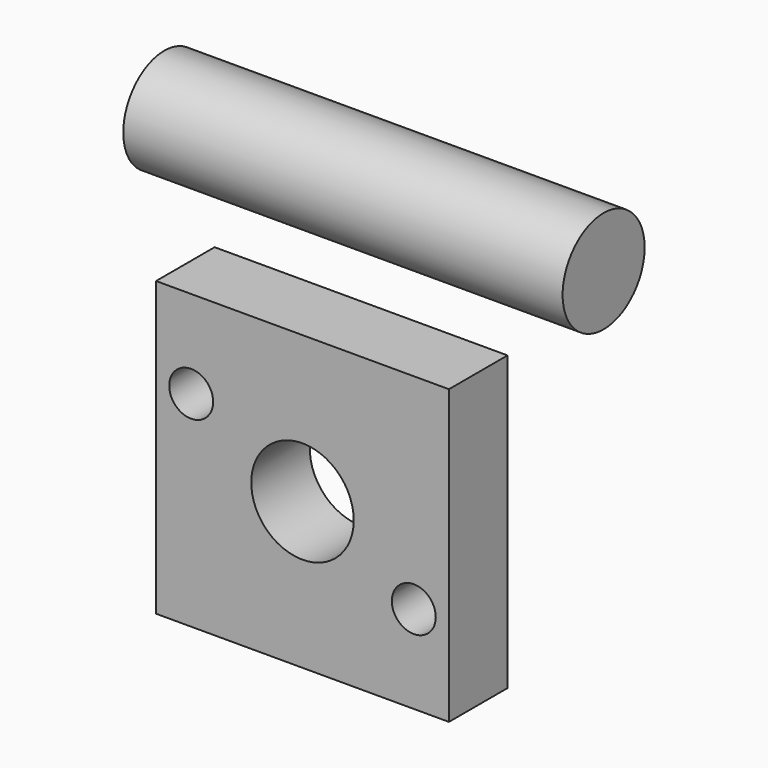
from build123d import *

# Parameters (mm, degrees)
F0_W     = 100
F0_H     = 100
F0_R     = 7.5
F0_R_2   = 17.5
F1_DEPTH = 25
F2_R     = 17.5
F3_DEPTH = 150
F4_R     = 7.5
F5_DEPTH = 5
F6_R     = 7.5
F7_DEPTH = 146.0218702087


with BuildPart() as f1:
    # F0 (on Front) → F1 (new body)
    with BuildSketch(Plane.XZ):
        Rectangle(F0_W, F0_H)
        with Locations((-38, -38)):
            Circle(F0_R, mode=Mode.SUBTRACT)
        with Locations((38, -38)):
            Circle(F0_R, mode=Mode.SUBTRACT)
        with Locations((-38, 38)):
            Circle(F0_R, mode=Mode.SUBTRACT)
        Circle(F0_R_2, mode=Mode.SUBTRACT)
        with Locations((38, 38)):
            Circle(F0_R, mode=Mode.SUBTRACT)
    extrude(amount=F1_DEPTH)

    # F4 (on face) → F5 (join)
    with BuildSketch(Plane.XZ.offset(25)):
        with Locations((-38, 38)):
            Circle(F4_R)
        with Locations((38, 38)):
            Circle(F4_R)
        with Locations((38, -38)):
            Circle(F4_R)
        with Locations((-38, -38)):
            Circle(F4_R)
    extrude(amount=-F5_DEPTH)

    # F6 (on face) → F7 (cut, through all)
    with BuildSketch(Plane.XZ.offset(25)):
        with Locations((-38, 20)):
            Circle(F6_R)
        with Locations((38, -20)):
            Circle(F6_R)
    extrude(amount=-F7_DEPTH, mode=Mode.SUBTRACT)


with BuildPart() as f3:
    # F2 (on Right) → F3 (new body)
    with BuildSketch(Plane.YZ):
        with Locations((103.5208702087, 16.9736910611)):
            Circle(F2_R)
    extrude(amount=-F3_DEPTH)


solid = Compound([f1.part, f3.part])
